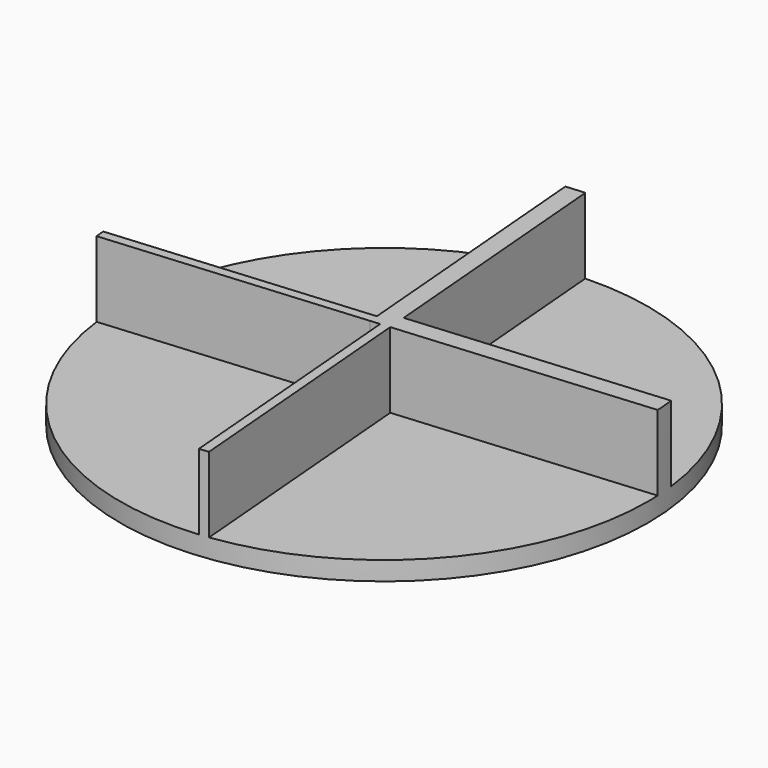
from build123d import *

# Parameters (mm, degrees)
F0_R     = 355.6
F1_DEPTH = 127
F3_DEPTH = 101.6


with BuildPart() as f1:
    # F0 (on Top) → F1 (new body)
    with BuildSketch(Plane.XY):
        Circle(F0_R)
    extrude(amount=F1_DEPTH)

    # F2 (on face) → F3 (cut)
    with BuildSketch(Plane.XY.offset(127)):
        with BuildLine():
            ThreePointArc((353.0999389591, 42.0926728434), (231.1027319808, 270.2644765244), (-13.2445388494, 355.353263937))
            Line((-13.2445388494, 355.353263937), (15.4660869459, 13.7182963842))
            Line((15.4660869459, 13.7182963842), (353.0999389591, 42.0926728434))
        make_face()
        with BuildLine():
            Line((-9.9109431068, 11.5856387734), (-38.6445388494, 353.4939315139))
            ThreePointArc((-38.6445388494, 353.4939315139), (-274.5766604834, 225.962425013), (-354.3236766316, -30.1013650562))
            Line((-354.3236766316, -30.1013650562), (-8.8475509302, -1.0679325675))
            Line((-8.8475509302, -1.0679325675), (-9.9109431068, 11.5856387734))
        make_face()
        with BuildLine():
            Line((33.6104931009, -354.0080433458), (4.9256574214, -12.679958877))
            Line((4.9256574214, -12.679958877), (-7.7819411742, -13.7478914444))
            Line((-7.7819411742, -13.7478914444), (-353.0195925051, -42.7612828101))
            ThreePointArc((-353.0195925051, -42.7612828101), (-222.9891918492, -276.9967153568), (33.6104931009, -354.0080433458))
        make_face()
        with BuildLine():
            Line((355.2049530963, 16.7571267176), (17.5950888785, -11.6152338337))
            Line((17.5950888785, -11.6152338337), (46.2493560151, -352.5795755119))
            ThreePointArc((46.2493560152, -352.5795755119), (267.2991124181, -234.5262128217), (355.6, 0))
            ThreePointArc((355.6, 0), (355.5012245556, 8.3808913292), (355.2049530963, 16.7571267176))
        make_face()
    extrude(amount=-F3_DEPTH, mode=Mode.SUBTRACT)


solid = f1.part
